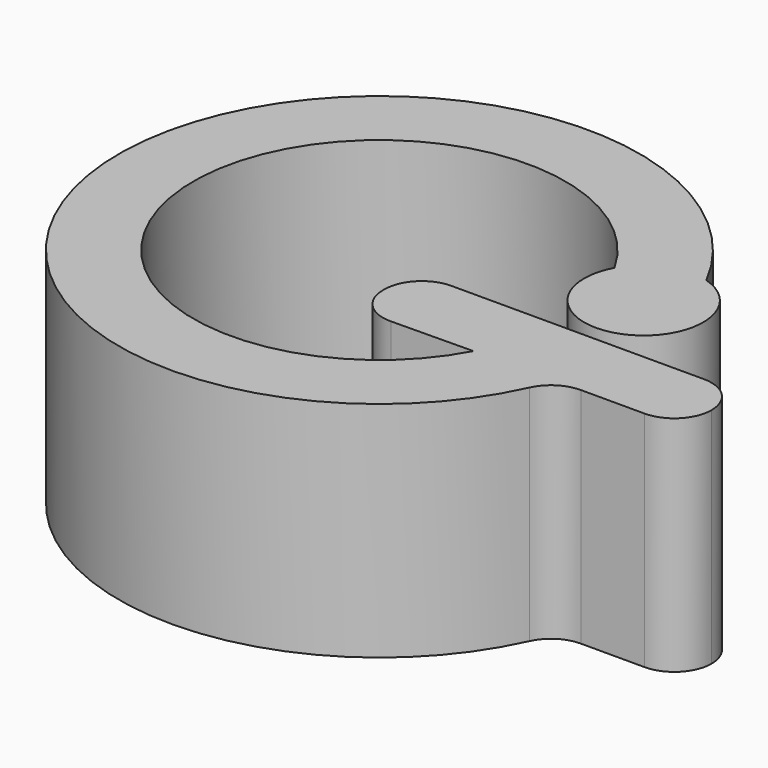
from build123d import *

# Parameters (mm, degrees)
F1_DEPTH = 6
F2_R     = 0.99999


# Not quite as in the source:
# - a fillet or chamfer is up to 0.001 mm smaller than in the source, because OpenCascade refuses the exact size


with BuildPart() as f1:
    # F0 (on Top) → F1 (new body)
    with BuildSketch(Plane.XY):
        with BuildLine():
            ThreePointArc((4.411359383, -2.3537009993), (-4.9996939131, -0.0553242752), (4.3581956764, 2.4507407954))
            ThreePointArc((4.3581956764, 2.4507407954), (6.3660027692, 0.1987741987), (6.2194307383, 3.2122704263))
            ThreePointArc((6.2194307383, 3.2122704263), (-6.9833792075, -0.482094228), (6.6018426545, -2.3271599784))
            Line((6.6018426545, -2.3271599784), (9.9892851541, -2.3271599784))
            Line((9.9892851541, -2.3271599784), (9.9892851541, -0.3271599784))
            Line((9.9892851541, -0.3271599784), (4.9892851541, -0.3271599784))
            Line((4.9892851541, -0.3271599784), (1.1988097103, -0.3271599784))
            Line((1.1988097103, -0.3271599784), (1.1988097103, -2.3926259018))
            Line((1.1988097103, -2.3926259018), (4.411359383, -2.3537009993))
        make_face()
    extrude(amount=F1_DEPTH)

    # F2 (radius 1 in the source; OpenCascade refuses exactly that, so slightly less here)
    f2_edges = [f1.edges().sort_by_distance(p)[0] for p in [
        (9.989285, -0.32716, 3),
        (1.19881, -0.32716, 3),
        (1.19881, -2.392626, 3),
        (9.989285, -2.32716, 3),
        (6.601843, -2.32716, 3),
    ]]
    fillet(f2_edges, radius=F2_R)


solid = f1.part
